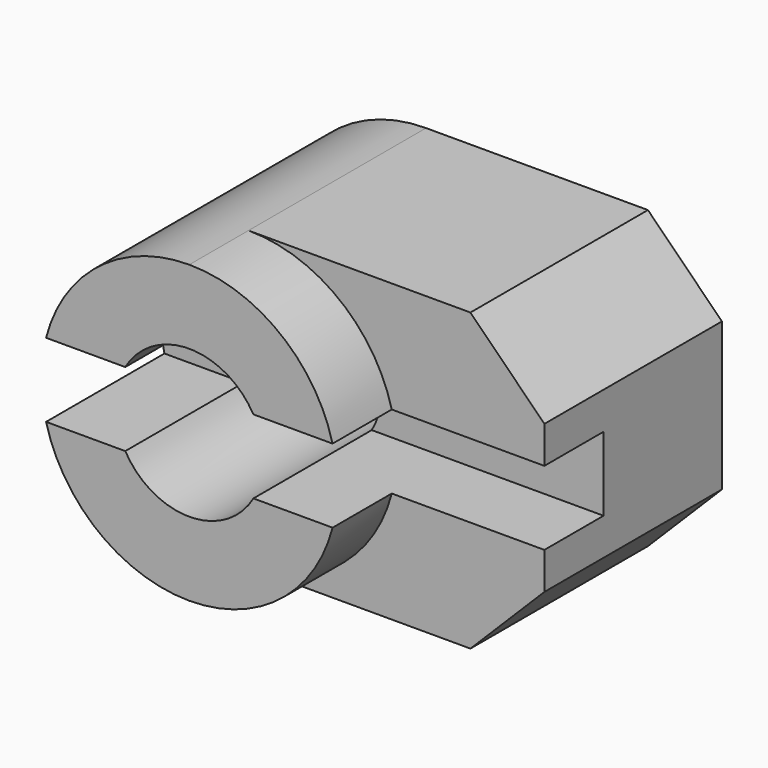
from build123d import *
from build123d import SkipClean  # not in build123d's __all__

# Parameters (mm, degrees)
F1_DEPTH = 20
F3_DEPTH = 50
F5_DEPTH = 5
F7_DEPTH = 25


# Not quite as in the source:
# - after a boolean that leaves OpenCascade's solid faulty, fix() repairs it


with BuildPart() as f1:
    # F0 (on Front) → F1 (new body)
    with BuildSketch(Plane.XZ):
        with BuildLine():
            ThreePointArc((0, -10), (7.0710678119, -7.0710678119), (10, 0))
            ThreePointArc((10, 0), (7.0710678119, 7.0710678119), (0, 10))
            ThreePointArc((0, 10), (-10, 0), (0, -10))
        make_face()
        with BuildLine():
            ThreePointArc((0, 10), (7.0710678119, 7.0710678119), (10, 0))
            ThreePointArc((10, 0), (7.0710678119, -7.0710678119), (0, -10))
            Line((0, -10), (15, -10))
            Line((15, -10), (20, -5))
            Line((20, -5), (20, 5))
            Line((20, 5), (15, 10))
            Line((15, 10), (0, 10))
        make_face()
    extrude(amount=F1_DEPTH)

    # F2 (on face) → F3 (cut)
    with BuildSketch(Plane.YZ.offset(20)):
        Polygon((-20, 2.5), (-20, 0), (-20, -2.5), (-10, -2.5), (-10, 2.5), align=None)
    extrude(amount=-F3_DEPTH, mode=Mode.SUBTRACT)

    # F4 (on face) → F5 (cut)
    with BuildSketch(Plane.XZ.offset(20)):
        with BuildLine():
            ThreePointArc((9.6824583655, -2.5), (6.123724357, -7.9056941504), (0, -10))
            Line((0, -10), (15, -10))
            Line((15, -10), (20, -5))
            Line((20, -5), (20, -2.5))
            Line((20, -2.5), (9.6824583655, -2.5))
        make_face()
        with BuildLine():
            Line((15, 10), (0, 10))
            ThreePointArc((0, 10), (6.123724357, 7.9056941504), (9.6824583655, 2.5))
            Line((9.6824583655, 2.5), (20, 2.5))
            Line((20, 2.5), (20, 5))
            Line((20, 5), (15, 10))
        make_face()
    with SkipClean():  # cleaning this boolean's faces spoils the solid; the shape is the same uncleaned
        extrude(amount=-F5_DEPTH, mode=Mode.SUBTRACT)

    # F6 (on face) → F7 (cut)
    with BuildSketch(Plane.XZ.offset(20)):
        with BuildLine():
            ThreePointArc((-4.3301270189, 2.5), (-1.2940952255, -4.8296291314), (5, 0))
            ThreePointArc((5, 0), (4.8296291314, 1.2940952255), (4.3301270189, 2.5))
            Line((4.3301270189, 2.5), (-4.3301270189, 2.5))
        make_face()
        with BuildLine():
            Line((-4.3301270189, 2.5), (4.3301270189, 2.5))
            ThreePointArc((4.3301270189, 2.5), (0, 5), (-4.3301270189, 2.5))
        make_face()
    extrude(amount=-F7_DEPTH, mode=Mode.SUBTRACT)

    add(f1.part.fix(), mode=Mode.REPLACE)


solid = f1.part
